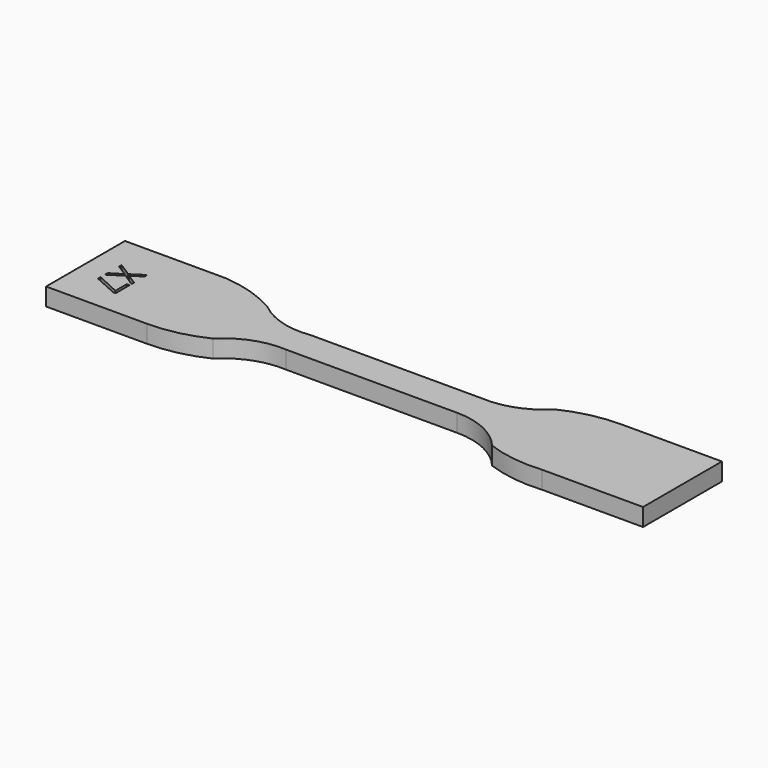
from build123d import *

# Parameters (mm, degrees)
F1_DEPTH     = 3.4
F2_TEXT_SIZE = 7.0564552314
F3_DEPTH     = 1


# Not quite as in the source:
# - Text() gives the source's letters only with a copy of the font that has no kerning and outlines rounded to 1/6400 em; it was checked with that copy


with BuildPart() as f1:
    # F0 (on Top) → F1 (new body)
    with BuildSketch(Plane.XY):
        with BuildLine():
            Line((-14.4320548165, 19.7811394548), (-33.8720548165, 19.7811394548))
            Line((-33.8720548165, 19.7811394548), (-33.8720548165, 0.7811394548))
            Line((-33.8720548165, 0.7811394548), (-14.4320548165, 0.7811394548))
            ThreePointArc((-14.4320548165, 0.7811394548), (-8.9053122052, 1.3996892086), (-3.6520548165, 3.2247301661))
            ThreePointArc((-3.6520548165, 3.2247301661), (1.3014698263, 6.4128780055), (7.1279451835, 7.2811394548))
            Line((7.1279451835, 7.2811394548), (40.1279451835, 7.2811394548))
            ThreePointArc((40.1279451835, 7.2811394548), (46.0837574042, 5.9511158081), (50.9079451835, 2.2137538538))
            ThreePointArc((50.9079451835, 2.2137538538), (56.2191047011, 0.9041953221), (61.6879451835, 0.7811394548))
            Line((61.6879451835, 0.7811394548), (81.1279451835, 0.7811394548))
            Line((81.1279451835, 0.7811394548), (81.1279451835, 19.7811394548))
            Line((81.1279451835, 19.7811394548), (61.6879451835, 19.7811394548))
            ThreePointArc((61.6879451835, 19.7811394548), (56.1612025723, 19.162589701), (50.9079451835, 17.3375487435))
            ThreePointArc((50.9079451835, 17.3375487435), (45.9544205407, 14.1494009041), (40.1279451835, 13.2811394548))
            Line((40.1279451835, 13.2811394548), (7.1279451835, 13.2811394548))
            ThreePointArc((7.1279451835, 13.2811394548), (1.4167452884, 13.6925537245), (-3.6520548165, 16.3560723447))
            ThreePointArc((-3.6520548165, 16.3560723447), (-8.8458057958, 18.686276846), (-14.4320548165, 19.7811394548))
        make_face()
    extrude(amount=F1_DEPTH)

    # F2 (on face) → F3 (cut)
    with BuildSketch(Plane.XY.offset(3.4)):
        with Locations(Location((-29.3720550835, 13.353464842), (0, 0, -90))):
            Text('X7', F2_TEXT_SIZE, font='Open Sans', text_align=(TextAlign.LEFT, TextAlign.BOTTOM))
    extrude(amount=-F3_DEPTH, mode=Mode.SUBTRACT)


solid = f1.part
